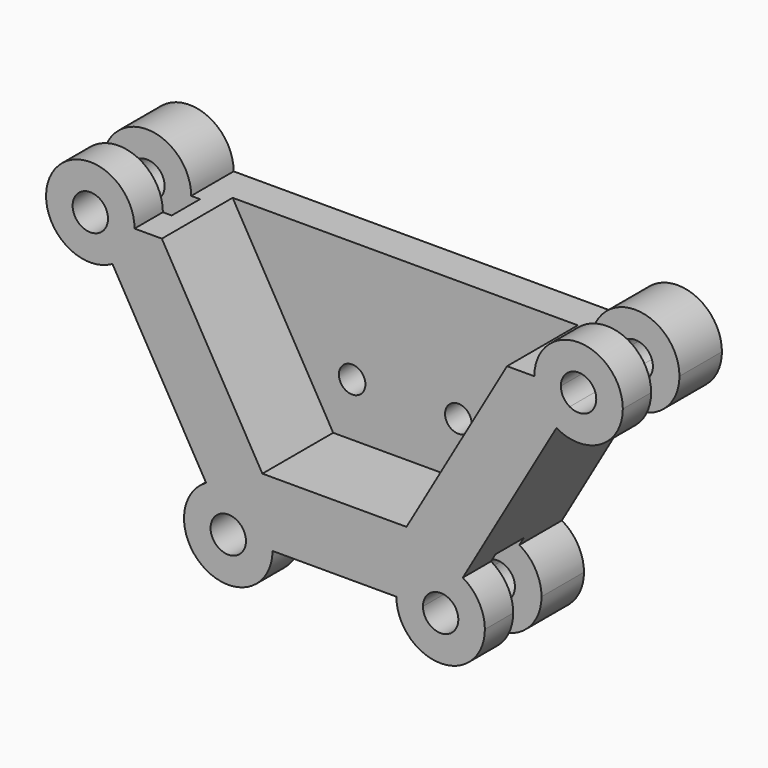
from build123d import *

# Parameters (mm, degrees)
F1_DEPTH  = 50.8
F3_DEPTH  = 76.2
F4_R      = 38.1
F1_FACE_R = 12.7
F5_DEPTH  = 12.7
F6_R      = 9.525
F7_DEPTH  = 25.401


with BuildPart() as f1:
    # F0 (on Front) → F1 (new body, symmetric)
    with BuildSketch(Plane.XZ):
        with BuildLine():
            ThreePointArc((-81.1352841451, 30.047498821), (-98.4838067731, 47.3960214491), (-74.7852841451, 41.0460214491))
            Line((-74.7852841451, 41.0460214491), (-55.7352841451, 41.0460214491))
            ThreePointArc((-55.7352841451, 41.0460214491), (-114.9815907152, 56.9210214491), (-71.6102841451, 13.5497148789))
            Line((-71.6102841451, 13.5497148789), (-81.1352841451, 30.047498821))
        make_face()
        with BuildLine():
            ThreePointArc((294.63812316, 41.0460214491), (262.88812316, 72.7960214491), (231.13812316, 41.0460214491))
            Line((231.13812316, 41.0460214491), (250.18812316, 41.0460214491))
            ThreePointArc((250.18812316, 41.0460214491), (262.88812316, 53.7460214491), (275.58812316, 41.0460214491))
            ThreePointArc((275.58812316, 41.0460214491), (269.23812316, 30.047498821), (256.53812316, 30.047498821))
            Line((256.53812316, 30.047498821), (247.01312316, 13.5497148789))
            ThreePointArc((247.01312316, 13.5497148789), (278.76312316, 13.5497148789), (294.63812316, 41.0460214491))
        make_face()
        with BuildLine():
            ThreePointArc((195.6514195075, -130.4039785509), (191.3977260776, -114.5289785509), (179.7764195075, -102.9076719808))
            Line((179.7764195075, -102.9076719808), (170.2514195075, -119.4054559229))
            ThreePointArc((170.2514195075, -119.4054559229), (174.8999421355, -124.0539785509), (176.6014195075, -130.4039785509))
            ThreePointArc((176.6014195075, -130.4039785509), (163.9014195075, -143.1039785509), (151.2014195075, -130.4039785509))
            Line((151.2014195075, -130.4039785509), (132.1514195075, -130.4039785509))
            ThreePointArc((132.1514195075, -130.4039785509), (163.9014195075, -162.1539785509), (195.6514195075, -130.4039785509))
        make_face()
        with BuildLine():
            Line((5.1514195075, -119.4054559229), (-4.3735804925, -102.9076719808))
            ThreePointArc((-4.3735804925, -102.9076719808), (-4.3735804925, -157.9002851211), (43.2514195075, -130.4039785509))
            Line((43.2514195075, -130.4039785509), (24.2014195075, -130.4039785509))
            ThreePointArc((24.2014195075, -130.4039785509), (5.1514195075, -141.402501179), (5.1514195075, -119.4054559229))
        make_face()
        with BuildLine():
            ThreePointArc((43.2514195075, -130.4039785509), (27.3764195075, -102.9076719808), (-4.3735804925, -102.9076719808))
            Line((-4.3735804925, -102.9076719808), (5.1514195075, -119.4054559229))
            ThreePointArc((5.1514195075, -119.4054559229), (17.8514195075, -119.4054559229), (24.2014195075, -130.4039785509))
            Line((24.2014195075, -130.4039785509), (43.2514195075, -130.4039785509))
        make_face()
        with BuildLine():
            Line((-55.7352841451, 41.0460214491), (-74.7852841451, 41.0460214491))
            ThreePointArc((-74.7852841451, 41.0460214491), (-76.486761517, 34.6960214491), (-81.1352841451, 30.047498821))
            Line((-81.1352841451, 30.047498821), (-71.6102841451, 13.5497148789))
            ThreePointArc((-71.6102841451, 13.5497148789), (-59.9889775749, 25.1710214491), (-55.7352841451, 41.0460214491))
        make_face()
        with BuildLine():
            Line((250.18812316, 41.0460214491), (231.13812316, 41.0460214491))
            ThreePointArc((231.13812316, 41.0460214491), (235.3918165899, 25.1710214491), (247.01312316, 13.5497148789))
            Line((247.01312316, 13.5497148789), (256.53812316, 30.047498821))
            ThreePointArc((256.53812316, 30.047498821), (251.889600532, 34.6960214491), (250.18812316, 41.0460214491))
        make_face()
        with BuildLine():
            Line((170.2514195075, -119.4054559229), (179.7764195075, -102.9076719808))
            ThreePointArc((179.7764195075, -102.9076719808), (148.0264195075, -102.9076719808), (132.1514195075, -130.4039785509))
            Line((132.1514195075, -130.4039785509), (151.2014195075, -130.4039785509))
            ThreePointArc((151.2014195075, -130.4039785509), (157.5514195075, -119.4054559229), (170.2514195075, -119.4054559229))
        make_face()
        with BuildLine():
            Line((231.13812316, 41.0460214491), (-55.7352841451, 41.0460214491))
            ThreePointArc((-55.7352841451, 41.0460214491), (-59.9889775749, 25.1710214491), (-71.6102841451, 13.5497148789))
            Line((-71.6102841451, 13.5497148789), (-4.3735804925, -102.9076719808))
            ThreePointArc((-4.3735804925, -102.9076719808), (27.3764195075, -102.9076719808), (43.2514195075, -130.4039785509))
            Line((43.2514195075, -130.4039785509), (132.1514195075, -130.4039785509))
            ThreePointArc((132.1514195075, -130.4039785509), (148.0264195075, -102.9076719808), (179.7764195075, -102.9076719808))
            Line((179.7764195075, -102.9076719808), (247.01312316, 13.5497148789))
            ThreePointArc((247.01312316, 13.5497148789), (235.3918165899, 25.1710214491), (231.13812316, 41.0460214491))
        make_face()
    extrude(amount=F1_DEPTH, both=True)

    # F2 (on face) → F3 (cut)
    with BuildSketch(Plane.XZ.offset(50.8)):
        Polygon((211.5616842291, 41.0460214491), (-36.1588452141, 41.0460214491), (36.0010718467, -83.9386211703), (139.4017671682, -83.9386211703), align=None)
    extrude(amount=-F3_DEPTH, mode=Mode.SUBTRACT)

    # F4 (on Front) + F1_face (on face) → F5 (cut, symmetric)
    with BuildSketch(Plane.XZ):
        with Locations((-87.4930471182, 41.0424880683)):
            Circle(F4_R)
        with Locations((262.2837722301, 41.0460214491)):
            Circle(F4_R)
        with Locations((163.9014195075, -130.4039785509)):
            Circle(F4_R)
        with Locations((11.5014195075, -130.4039785509)):
            Circle(F4_R)
    with BuildSketch(Plane(origin=(87.7014195075, -50.8, -33.7225685026), x_dir=(1, 0, 0), z_dir=(0, -1, 0))):
        with BuildLine():
            Line((-123.8602647216, 74.7685899517), (-143.4367036526, 74.7685899517))
            ThreePointArc((-143.4367036526, 74.7685899517), (-202.6830102227, 90.6435899517), (-159.3117036526, 47.2722833815))
            Line((-159.3117036526, 47.2722833815), (-92.075, -69.1851034782))
            ThreePointArc((-92.075, -69.1851034782), (-92.075, -124.1777166185), (-44.45, -96.6814100483))
            Line((-44.45, -96.6814100483), (44.45, -96.6814100483))
            ThreePointArc((44.45, -96.6814100483), (92.075, -124.1777166185), (92.075, -69.1851034782))
            Line((92.075, -69.1851034782), (159.3117036526, 47.2722833815))
            ThreePointArc((159.3117036526, 47.2722833815), (202.6830102227, 90.6435899517), (143.4367036526, 74.7685899517))
            Line((143.4367036526, 74.7685899517), (123.8602647216, 74.7685899517))
            Line((123.8602647216, 74.7685899517), (51.7003476608, -50.2160526677))
            Line((51.7003476608, -50.2160526677), (-51.7003476608, -50.2160526677))
            Line((-51.7003476608, -50.2160526677), (-123.8602647216, 74.7685899517))
        make_face()
        with Locations((-76.2, -96.6814100483)):
            Circle(F1_FACE_R, mode=Mode.SUBTRACT)
        with Locations((76.2, -96.6814100483)):
            Circle(F1_FACE_R, mode=Mode.SUBTRACT)
        with Locations((-175.1867036526, 74.7685899517)):
            Circle(F1_FACE_R, mode=Mode.SUBTRACT)
        with Locations((175.1867036526, 74.7685899517)):
            Circle(F1_FACE_R, mode=Mode.SUBTRACT)
    extrude(amount=F5_DEPTH, both=True, mode=Mode.SUBTRACT)

    # F6 (on face) → F7 (cut, through all)
    with BuildSketch(Plane.XZ.offset(-25.4)):
        with Locations((49.6014195075, -45.8386211703)):
            Circle(F6_R)
        with Locations((125.8014195075, -45.8386211703)):
            Circle(F6_R)
    extrude(amount=-F7_DEPTH, mode=Mode.SUBTRACT)


solid = f1.part
